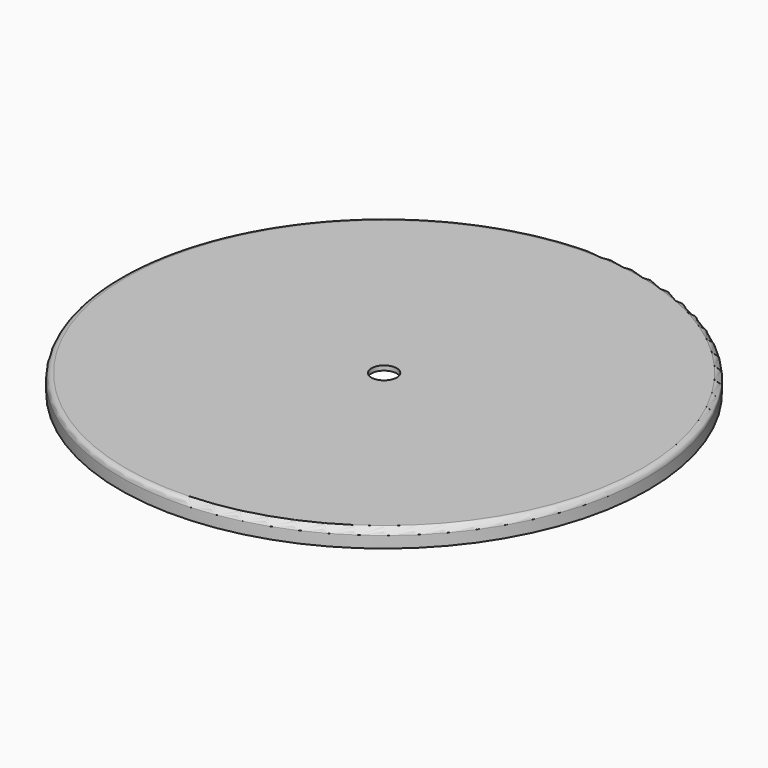
from build123d import *

# Parameters (mm, degrees)
F0_R     = 91.6
F1_DEPTH = 6
F2_R     = 2
F3_T     = -1.6
F6_R     = 30
F7_DEPTH = 50
F8_R     = 26.5
F9_DEPTH = 56.001
F12_D    = 8.8


with BuildPart() as f1:
    # F0 (on Top) → F1 (new body)
    with BuildSketch(Plane.XY):
        Circle(F0_R)
    extrude(amount=F1_DEPTH)

    # F2
    f2_edges = [f1.edges().sort_by_distance(p)[0] for p in [
        (-91.6, 0, 6),
    ]]
    fillet(f2_edges, radius=F2_R)

    # F3
    f3_openings = [f1.faces().sort_by_distance(p)[0] for p in [
        (0, 0, 0),
    ]]
    offset(amount=F3_T, openings=f3_openings)


with BuildPart() as f5_1:
    # F5: copy of F1
    add(f1.part)


with BuildPart() as f7:
    # F6 (on face) → F7 (new body)
    with BuildSketch(Plane.XY.offset(6)):
        Circle(F6_R)
    extrude(amount=F7_DEPTH)

    # F8 (on face) → F9 (cut, through all)
    with BuildSketch(Plane.XY.offset(56)):
        Circle(F8_R)
    extrude(amount=-F9_DEPTH, mode=Mode.SUBTRACT)


with BuildPart() as f1_1:
    add(f1.part)

    # F12 (through all)
    with Locations(Plane.XY.offset(6)):
        with Locations((0, 0)):
            Hole(F12_D / 2)


solid = f1_1.part
